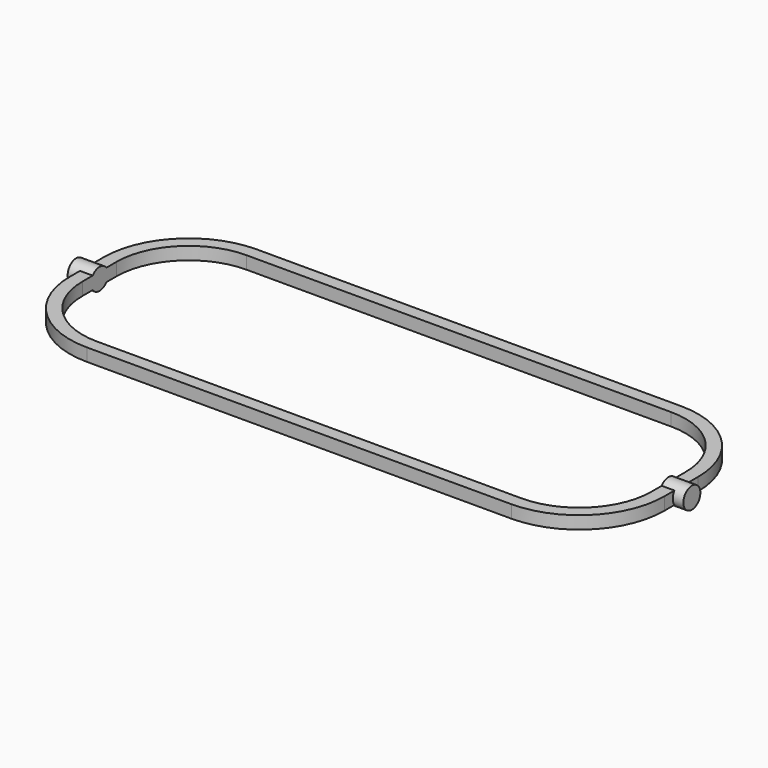
from build123d import *

# Parameters (mm, degrees)
F1_DEPTH = 1.5
F2_R     = 2.5
F3_DEPTH = 72.5
F4_DEPTH = 67


with BuildPart() as f1:
    # F0 (on Top) → F1 (new body, symmetric)
    with BuildSketch(Plane.XY):
        with BuildLine():
            Line((50, 25), (-50, 25))
            ThreePointArc((-50, 25), (-64.1421356237, 19.1421356237), (-70, 5))
            Line((-70, 5), (-70, -5))
            ThreePointArc((-70, -5), (-64.1421356237, -19.1421356237), (-50, -25))
            Line((-50, -25), (50, -25))
            ThreePointArc((50, -25), (64.1421356237, -19.1421356237), (70, -5))
            Line((70, -5), (70, 5))
            ThreePointArc((70, 5), (64.1421356237, 19.1421356237), (50, 25))
        make_face()
        with BuildLine():
            Line((-67, -5), (-67, 5))
            ThreePointArc((-67, 5), (-62.0208152802, 17.0208152802), (-50, 22))
            Line((-50, 22), (50, 22))
            ThreePointArc((50, 22), (62.0208152802, 17.0208152802), (67, 5))
            Line((67, 5), (67, -5))
            ThreePointArc((67, -5), (62.0208152802, -17.0208152802), (50, -22))
            Line((50, -22), (-50, -22))
            ThreePointArc((-50, -22), (-62.0208152802, -17.0208152802), (-67, -5))
        make_face(mode=Mode.SUBTRACT)
    extrude(amount=F1_DEPTH, both=True)

    # F2 (on Right) → F3 (join)
    with BuildSketch(Plane.YZ):
        Circle(F2_R)
    extrude(amount=F3_DEPTH)

    # F2 (on Right) → F4 (cut, through all)
    with BuildSketch(Plane.YZ):
        Circle(F2_R)
    extrude(amount=F4_DEPTH, mode=Mode.SUBTRACT)

    # F5: F1 across plane


with BuildPart() as f1_1:
    add(f1.part)
    add(f1.part.mirror(Plane.YZ))


solid = f1_1.part
